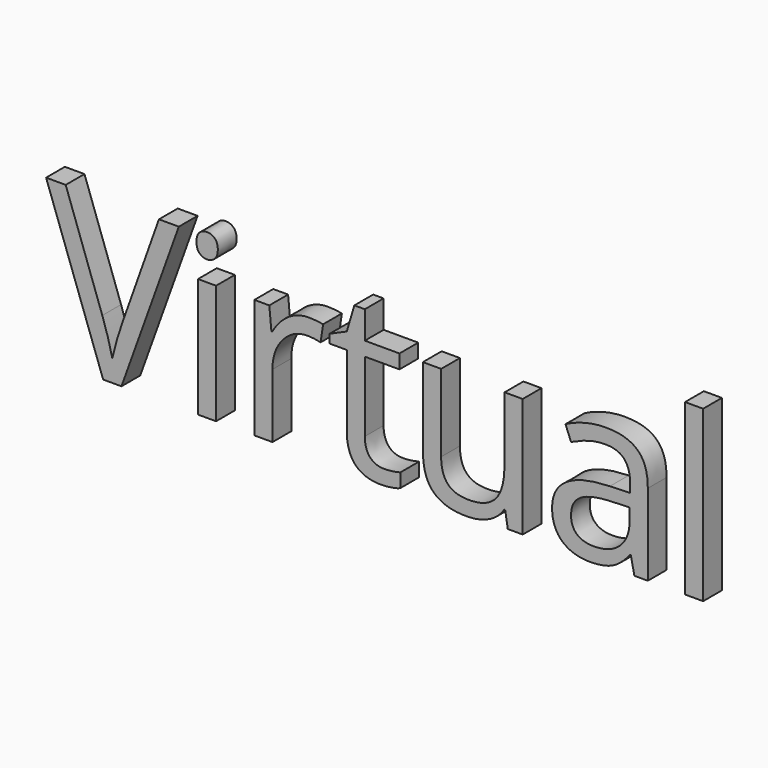
from build123d import *

# Parameters (mm, degrees)
F0_TEXT_SIZE = 120.5737702549
F1_DEPTH     = 12.7


# Not quite as in the source:
# - Text() gives the source's letters only with a copy of the font that has no kerning and outlines rounded to 1/6400 em; it was checked with that copy


with BuildPart() as f1:
    # F0 (on Front) → F1 (new body)
    with BuildSketch(Plane.XZ):
        with Locations((-46.7609837651, -44.564768672)):
            Text('Virtual', F0_TEXT_SIZE, font='Open Sans', text_align=(TextAlign.LEFT, TextAlign.BOTTOM))
    extrude(amount=F1_DEPTH)


solid = f1.part
